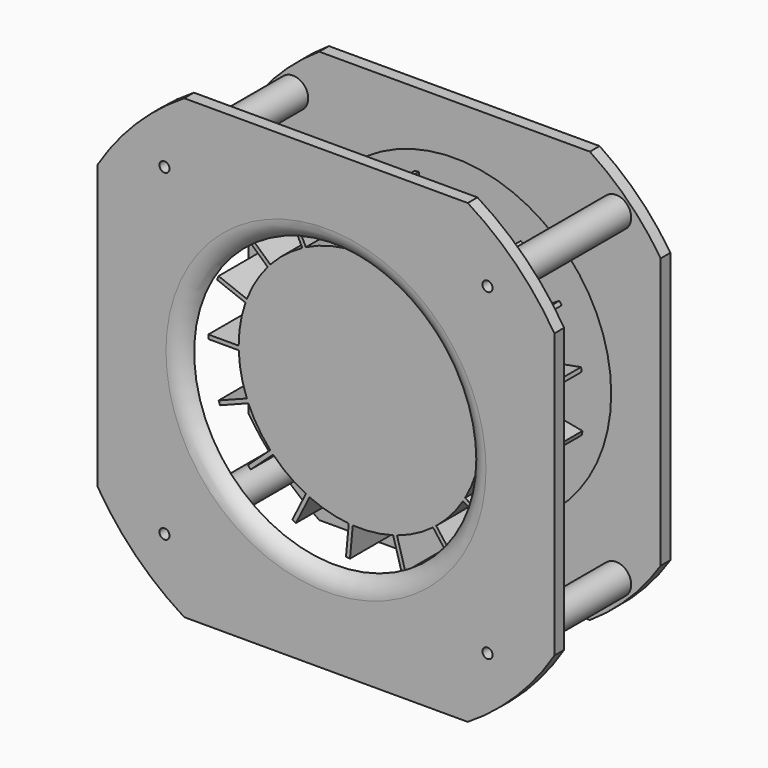
from build123d import *

# Parameters (mm, degrees)
F0_R      = 2.5
F0_R_2    = 70
F1_DEPTH  = 6
F3_R      = 77.5
F4_DEPTH  = 6
F5_R      = 7.5
F5_R_2    = 2.5
F6_DEPTH  = 73.5
F9_DEPTH  = 45
F11_R     = 35
F12_DEPTH = 32.5
F13_R     = 91.0184628647
F13_R_2   = 34.9752900341
F14_DEPTH = 8
F15_SIZE  = 4.99999
F13_R_3   = 77.5
F17_DEPTH = 25


# Not quite as in the source:
# - a fillet or chamfer that OpenCascade refuses, or shapes differently, is made with other operations: its cross-section is extruded or revolved along the edge and cut away or added
# - a fillet or chamfer is up to 0.001 mm smaller than in the source, because OpenCascade refuses the exact size


with BuildPart() as f1:
    # F0 (on Front) → F1 (new body)
    with BuildSketch(Plane.XZ):
        with BuildLine():
            Line((70.142711667, 113), (-70.142711667, 113))
            ThreePointArc((-70.142711667, 113), (-94.0452018978, 94.0452018978), (-113, 70.142711667))
            Line((-113, 70.142711667), (-113, -70.142711667))
            ThreePointArc((-113, -70.142711667), (-94.0452018978, -94.0452018978), (-70.142711667, -113))
            Line((-70.142711667, -113), (70.142711667, -113))
            ThreePointArc((70.142711667, -113), (94.0452018978, -94.0452018978), (113, -70.142711667))
            Line((113, -70.142711667), (113, 70.142711667))
            ThreePointArc((113, 70.142711667), (94.0452018978, 94.0452018978), (70.142711667, 113))
        make_face()
        with Locations((-79.9030662741, -79.9030662741)):
            Circle(F0_R, mode=Mode.SUBTRACT)
        with Locations((79.9030662741, -79.9030662741)):
            Circle(F0_R, mode=Mode.SUBTRACT)
        with Locations((-79.9030662741, 79.9030662741)):
            Circle(F0_R, mode=Mode.SUBTRACT)
        Circle(F0_R_2, mode=Mode.SUBTRACT)
        with Locations((79.9030662741, 79.9030662741)):
            Circle(F0_R, mode=Mode.SUBTRACT)
    extrude(amount=-F1_DEPTH)



with BuildPart() as f4:
    # F3 (on offset) → F4 (new body)
    with BuildSketch(Plane(origin=(0, 85.5, 0), x_dir=(-1, 0, 0), z_dir=(0, 1, 0))):
        with BuildLine():
            Line((102, -66.9328021227), (102, 66.9328021227))
            ThreePointArc((102, 66.9328021227), (86.2670273048, 86.2670273048), (66.9328021227, 102))
            Line((66.9328021227, 102), (-66.9328021227, 102))
            ThreePointArc((-66.9328021227, 102), (-86.2670273048, 86.2670273048), (-102, 66.9328021227))
            Line((-102, 66.9328021227), (-102, -66.9328021227))
            ThreePointArc((-102, -66.9328021227), (-86.2670273048, -86.2670273048), (-66.9328021227, -102))
            Line((-66.9328021227, -102), (66.9328021227, -102))
            ThreePointArc((66.9328021227, -102), (86.2670273048, -86.2670273048), (102, -66.9328021227))
        make_face()
        Circle(F3_R, mode=Mode.SUBTRACT)
    extrude(amount=-F4_DEPTH)


with BuildPart() as f1_1:
    add(f1.part)

    add(f4.part)  # F6 merges F4
    # F5 (on face) → F6 (join, through all)
    with BuildSketch(Plane(origin=(0, 6, 0), x_dir=(-1, 0, 0), z_dir=(0, 1, 0))):
        with Locations((-79.9030662741, 79.9030662741)):
            Circle(F5_R)
        with Locations((-79.9030662741, 79.9030662741)):
            Circle(F5_R_2, mode=Mode.SUBTRACT)
        with Locations((79.9030662741, 79.9030662741)):
            Circle(F5_R)
        with Locations((79.9030662741, 79.9030662741)):
            Circle(F5_R_2, mode=Mode.SUBTRACT)
        with Locations((-79.9030662741, -79.9030662741)):
            Circle(F5_R)
        with Locations((-79.9030662741, -79.9030662741)):
            Circle(F5_R_2, mode=Mode.SUBTRACT)
        with Locations((79.9030662741, -79.9030662741)):
            Circle(F5_R)
        with Locations((79.9030662741, -79.9030662741)):
            Circle(F5_R_2, mode=Mode.SUBTRACT)
    extrude(amount=F6_DEPTH)



with BuildPart() as f9:
    # F8 (on offset) → F9 (new body)
    with BuildSketch(Plane(origin=(0, 21, 0), x_dir=(-1, 0, 0), z_dir=(0, 1, 0))):
        with BuildLine():
            Line((59.9666574023, -2), (60, 0))
            ThreePointArc((60, 0), (59.1539667436, 10.0403296009), (56.6397260502, 19.7975107769))
            ThreePointArc((56.6397260502, 19.7975107769), (56.3018523257, 20.7388867757), (55.9483337643, 21.6744999712))
            ThreePointArc((55.9483337643, 21.6744999712), (51.5324458534, 30.7312060349), (45.6632858435, 38.9212580215))
            ThreePointArc((45.6632858435, 38.9212580215), (45.008163744, 39.6770109307), (44.3405350332, 40.4217386188))
            ThreePointArc((44.3405350332, 40.4217386188), (36.9511825996, 47.2716628065), (28.5197658546, 52.7884737002))
            ThreePointArc((28.5197658546, 52.7884737002), (27.6358732499, 53.2565349015), (26.7443013466, 53.7097974813))
            ThreePointArc((26.7443013466, 53.7097974813), (17.3794573821, 57.4278195747), (7.5244934536, 59.5263134947))
            ThreePointArc((7.5244934536, 59.5263134947), (6.5312049376, 59.6434687293), (5.5361015678, 59.7440505777))
            ThreePointArc((5.5361015678, 59.7440505777), (-4.5394598577, 59.8280310908), (-14.487003483, 58.224794805))
            ThreePointArc((-14.487003483, 58.224794805), (-15.455538792, 57.9752216093), (-16.4197794043, 57.7095385904))
            ThreePointArc((-16.4197794043, 57.7095385904), (-25.8452978897, 54.1481354895), (-34.5419503239, 49.0596949422))
            ThreePointArc((-34.5419503239, 49.0596949422), (-35.3549263658, 48.4770995592), (-36.1580781828, 47.8810336368))
            ThreePointArc((-36.1580781828, 47.8810336368), (-43.660585228, 41.1552341452), (-49.9318153701, 33.2688114283))
            ThreePointArc((-49.9318153701, 33.2688114283), (-50.4794352254, 32.4318765927), (-51.0130281438, 31.5859297726))
            ThreePointArc((-51.0130281438, 31.5859297726), (-55.5792685996, 22.6040903806), (-58.5781120687, 12.9847905821))
            ThreePointArc((-58.5781120687, 12.9847905821), (-58.7864166416, 12.0065489812), (-58.978385981, 11.024971069))
            ThreePointArc((-58.978385981, 11.024971069), (-59.9916637715, 1.0001389564), (-59.31311014, -9.0528981834))
            ThreePointArc((-59.31311014, -9.0528981834), (-59.1539667436, -10.0403296009), (-58.978385981, -11.024971069))
            ThreePointArc((-58.978385981, -11.024971069), (-56.3018523257, -20.7388867757), (-52.0375440216, -29.8679428853))
            ThreePointArc((-52.0375440216, -29.8679428853), (-51.5324458534, -30.7312060349), (-51.0130281438, -31.5859297726))
            ThreePointArc((-51.0130281438, -31.5859297726), (-45.008163744, -39.6770109307), (-37.7340192331, -46.6491563967))
            ThreePointArc((-37.7340192331, -46.6491563967), (-36.9511825996, -47.2716628065), (-36.1580781828, -47.8810336368))
            ThreePointArc((-36.1580781828, -47.8810336368), (-27.6358732499, -53.2565349015), (-18.3343060557, -57.1301428447))
            ThreePointArc((-18.3343060557, -57.1301428447), (-17.3794573821, -57.4278195747), (-16.4197794043, -57.7095385904))
            ThreePointArc((-16.4197794043, -57.7095385904), (-6.5312049376, -59.6434687293), (3.5415567484, -59.8953869325))
            ThreePointArc((3.5415567484, -59.8953869325), (4.5394598577, -59.8280310908), (5.5361015678, -59.7440505777))
            ThreePointArc((5.5361015678, -59.7440505777), (15.455538792, -57.9752216093), (24.9391126892, -54.5714271233))
            ThreePointArc((24.9391126892, -54.5714271233), (25.8452978897, -54.1481354895), (26.7443013466, -53.7097974813))
            ThreePointArc((26.7443013466, -53.7097974813), (35.3549263658, -48.4770995592), (42.9685032689, -41.8772936904))
            ThreePointArc((42.9685032689, -41.8772936904), (43.660585228, -41.1552341452), (44.3405350332, -40.4217386188))
            ThreePointArc((44.3405350332, -40.4217386188), (50.4794352254, -32.4318765927), (55.1947593854, -23.5273996945))
            ThreePointArc((55.1947593854, -23.5273996945), (55.5792685996, -22.6040903806), (55.9483337643, -21.6744999712))
            ThreePointArc((55.9483337643, -21.6744999712), (58.7864166416, -12.0065489812), (59.9666574023, -2))
        make_face()
        with BuildLine():
            Line((75, 0), (60, 0))
            ThreePointArc((60, 0), (59.9916637715, -1.0001389564), (59.9666574023, -2))
            Line((59.9666574023, -2), (75, -2))
            Line((75, -2), (75, 0))
        make_face()
        with BuildLine():
            ThreePointArc((59.9666574023, -2), (59.9916637715, -1.0001389564), (60, 0))
            Line((60, 0), (59.9666574023, -2))
        make_face()
        with BuildLine():
            ThreePointArc((55.9483337643, 21.6744999712), (56.3018523257, 20.7388867757), (56.6397260502, 19.7975107769))
            Line((56.6397260502, 19.7975107769), (70.6579005377, 25.2281805052))
            Line((70.6579005377, 25.2281805052), (69.9354172053, 27.093124964))
            Line((69.9354172053, 27.093124964), (55.9483337643, 21.6744999712))
        make_face()
        with BuildLine():
            Line((69.9354172053, -27.093124964), (55.9483337643, -21.6744999712))
            ThreePointArc((55.9483337643, -21.6744999712), (55.5792685996, -22.6040903806), (55.1947593854, -23.5273996945))
            Line((55.1947593854, -23.5273996945), (69.212933873, -28.9580694228))
            Line((69.212933873, -28.9580694228), (69.9354172053, -27.093124964))
        make_face()
        with BuildLine():
            ThreePointArc((44.3405350332, 40.4217386188), (45.008163744, 39.6770109307), (45.6632858435, 38.9212580215))
            Line((45.6632858435, 38.9212580215), (56.7730600788, 49.0491554391))
            Line((56.7730600788, 49.0491554391), (55.4256687915, 50.5271732735))
            Line((55.4256687915, 50.5271732735), (44.3405350332, 40.4217386188))
        make_face()
        with BuildLine():
            Line((55.4256687915, -50.5271732735), (44.3405350332, -40.4217386188))
            ThreePointArc((44.3405350332, -40.4217386188), (43.660585228, -41.1552341452), (42.9685032689, -41.8772936904))
            Line((42.9685032689, -41.8772936904), (54.0782775043, -52.0051911079))
            Line((54.0782775043, -52.0051911079), (55.4256687915, -50.5271732735))
        make_face()
        with BuildLine():
            ThreePointArc((26.7443013466, 53.7097974813), (27.6358732499, 53.2565349015), (28.5197658546, 52.7884737002))
            Line((28.5197658546, 52.7884737002), (35.220703266, 66.2457701401))
            Line((35.220703266, 66.2457701401), (33.4303766832, 67.1372468516))
            Line((33.4303766832, 67.1372468516), (26.7443013466, 53.7097974813))
        make_face()
        with BuildLine():
            Line((33.4303766832, -67.1372468516), (26.7443013466, -53.7097974813))
            ThreePointArc((26.7443013466, -53.7097974813), (25.8452978897, -54.1481354895), (24.9391126892, -54.5714271233))
            Line((24.9391126892, -54.5714271233), (31.6400501005, -68.0287235632))
            Line((31.6400501005, -68.0287235632), (33.4303766832, -67.1372468516))
        make_face()
        with BuildLine():
            ThreePointArc((5.5361015678, 59.7440505777), (6.5312049376, 59.6434687293), (7.5244934536, 59.5263134947))
            Line((7.5244934536, 59.5263134947), (8.9115953123, 74.4955265032))
            Line((8.9115953123, 74.4955265032), (6.9201269597, 74.6800632221))
            Line((6.9201269597, 74.6800632221), (5.5361015678, 59.7440505777))
        make_face()
        with BuildLine():
            Line((6.9201269597, -74.6800632221), (5.5361015678, -59.7440505777))
            ThreePointArc((5.5361015678, -59.7440505777), (4.5394598577, -59.8280310908), (3.5415567484, -59.8953869325))
            Line((3.5415567484, -59.8953869325), (4.9286586072, -74.8645999411))
            Line((4.9286586072, -74.8645999411), (6.9201269597, -74.6800632221))
        make_face()
        with BuildLine():
            ThreePointArc((-16.4197794043, 57.7095385904), (-15.455538792, 57.9752216093), (-14.487003483, 58.224794805))
            Line((-14.487003483, 58.224794805), (-18.6010729691, 72.6842492181))
            Line((-18.6010729691, 72.6842492181), (-20.5247242554, 72.136923238))
            Line((-20.5247242554, 72.136923238), (-16.4197794043, 57.7095385904))
        make_face()
        with BuildLine():
            Line((-20.5247242554, -72.136923238), (-16.4197794043, -57.7095385904))
            ThreePointArc((-16.4197794043, -57.7095385904), (-17.3794573821, -57.4278195747), (-18.3343060557, -57.1301428447))
            Line((-18.3343060557, -57.1301428447), (-22.4483755418, -71.5895972578))
            Line((-22.4483755418, -71.5895972578), (-20.5247242554, -72.136923238))
        make_face()
        with BuildLine():
            ThreePointArc((-36.1580781828, 47.8810336368), (-35.3549263658, 48.4770995592), (-34.5419503239, 49.0596949422))
            Line((-34.5419503239, 49.0596949422), (-43.6015632739, 61.0565613188))
            Line((-43.6015632739, 61.0565613188), (-45.1975977284, 59.851292046))
            Line((-45.1975977284, 59.851292046), (-36.1580781828, 47.8810336368))
        make_face()
        with BuildLine():
            Line((-45.1975977284, -59.851292046), (-36.1580781828, -47.8810336368))
            ThreePointArc((-36.1580781828, -47.8810336368), (-36.9511825996, -47.2716628065), (-37.7340192331, -46.6491563967))
            Line((-37.7340192331, -46.6491563967), (-46.793632183, -58.6460227733))
            Line((-46.793632183, -58.6460227733), (-45.1975977284, -59.851292046))
        make_face()
        with BuildLine():
            ThreePointArc((-51.0130281438, 31.5859297726), (-50.4794352254, 32.4318765927), (-49.9318153701, 33.2688114283))
            Line((-49.9318153701, 33.2688114283), (-62.713420854, 41.1828464873))
            Line((-62.713420854, 41.1828464873), (-63.7662851797, 39.4824122158))
            Line((-63.7662851797, 39.4824122158), (-51.0130281438, 31.5859297726))
        make_face()
        with BuildLine():
            Line((-63.7662851797, -39.4824122158), (-51.0130281438, -31.5859297726))
            ThreePointArc((-51.0130281438, -31.5859297726), (-51.5324458534, -30.7312060349), (-52.0375440216, -29.8679428853))
            Line((-52.0375440216, -29.8679428853), (-64.8191495055, -37.7819779443))
            Line((-64.8191495055, -37.7819779443), (-63.7662851797, -39.4824122158))
        make_face()
        with BuildLine():
            ThreePointArc((-58.978385981, 11.024971069), (-58.7864166416, 12.0065489812), (-58.5781120687, 12.9847905821))
            Line((-58.5781120687, 12.9847905821), (-73.3554834407, 15.7471600356))
            Line((-73.3554834407, 15.7471600356), (-73.7229824763, 13.7812138362))
            Line((-73.7229824763, 13.7812138362), (-58.978385981, 11.024971069))
        make_face()
        with BuildLine():
            Line((-73.7229824763, -13.7812138362), (-58.978385981, -11.024971069))
            ThreePointArc((-58.978385981, -11.024971069), (-59.1539667436, -10.0403296009), (-59.31311014, -9.0528981834))
            Line((-59.31311014, -9.0528981834), (-74.0904815119, -11.8152676369))
            Line((-74.0904815119, -11.8152676369), (-73.7229824763, -13.7812138362))
        make_face()
    extrude(amount=F9_DEPTH)

    # F11 (on offset) → F12 (join, through all)
    with BuildSketch(Plane.XZ.offset(-98.5)):
        Circle(F11_R)
    extrude(amount=F12_DEPTH)


with BuildPart() as f1_2:
    add(f1_1.part)

    add(f9.part)  # F14 merges F9
    # F13 (on face) → F14 (join)
    with BuildSketch(Plane(origin=(0, 85.5, 0), x_dir=(-1, 0, 0), z_dir=(0, 1, 0))):
        Circle(F13_R)
        Circle(F13_R_2, mode=Mode.SUBTRACT)
    extrude(amount=F14_DEPTH)

    # F15 (size 5 in the source; OpenCascade refuses exactly that, so slightly less here)
    f15_edges = [f1_2.edges().sort_by_distance(p)[0] for p in [
        (91.018463, 93.5, 0),
        (-35, 98.5, 0),
    ]]
    chamfer(f15_edges, length=F15_SIZE)

    # F16: fillet of radius 10 on 1 edges, made by hand

    # F16_s1 → F16_t2 (revolve, cut)
    with BuildSketch(Plane.XY):
        with BuildLine():
            ThreePointArc((70, 6), (73.6879258149, 1.6333997347), (79.1651513899, 0))
            Line((79.1651513899, 0), (70, 0))
            Line((70, 0), (70, 6))
        make_face()
    revolve(axis=Axis((0, 0, 0), (0, -1, 0)), mode=Mode.SUBTRACT)


with BuildPart() as f17:
    # F13 (on face) → F17 (new body)
    with BuildSketch(Plane(origin=(0, 85.5, 0), x_dir=(-1, 0, 0), z_dir=(0, 1, 0))):
        Circle(F13_R)
        Circle(F13_R_3, mode=Mode.SUBTRACT)
        Circle(F13_R_3)
        Circle(F13_R_2, mode=Mode.SUBTRACT)
    extrude(amount=F17_DEPTH)


solid = f1_2.part
